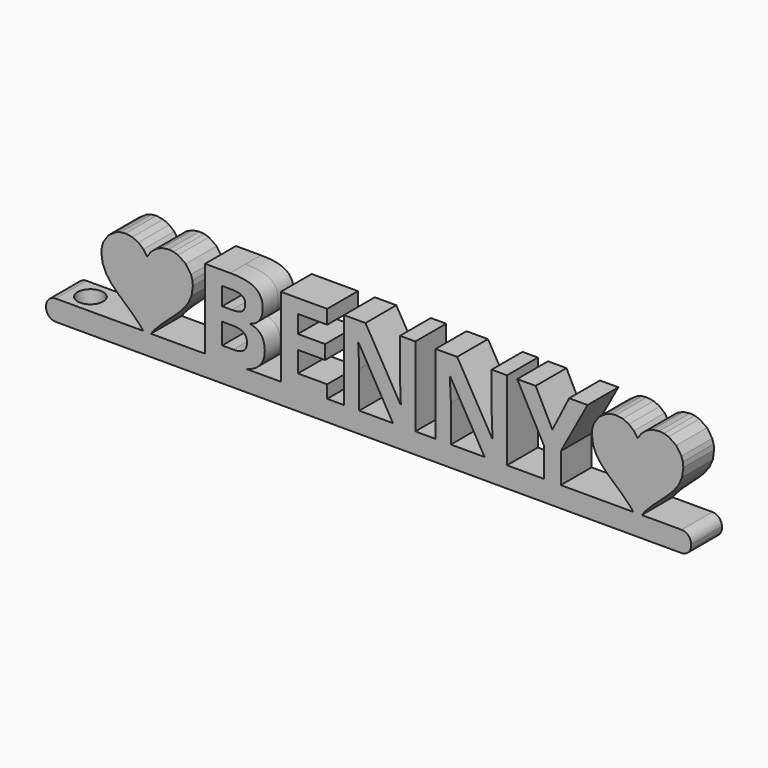
from build123d import *

# Parameters (mm, degrees)
F0_TEXT_SIZE = 17.5671771164
F1_DEPTH     = 3
F2_W         = 93
F2_H         = 6
F3_DEPTH     = 0.2
F4_DEPTH     = 3
F5_W         = 6
F5_H         = 3.2
F6_DEPTH     = 7.5
F7_R         = 1.5
F8_R         = 2
F9_DEPTH     = 4
F10_R        = 1.5


# Not quite as in the source:
# - Text() gives the source's letters only with a copy of the font that has no kerning and outlines rounded to 1/6400 em; it was checked with that copy


with BuildPart() as f1:
    # F0 (on Front) → F1 (new body, symmetric)
    with BuildSketch(Plane.XZ):
        Polygon((61.1623563837, 12.4433699982), (60.1013363837, 12.5970599982), (59.3427263837, 12.5204799982), (58.6359263837, 12.3008699982), (57.4385863837, 11.4933499982), (56.6309663837, 10.2961199982), (56.4113163837, 9.5893599982), (56.3347263837, 8.8307599982), (56.5232463837, 7.3860999982), (57.0439863837, 6.1597099982), (57.8297363837, 5.0814099982), (58.8132663837, 4.0810299982), (61.1101163837, 2.0250499982), (62.2947063837, 0.8247399982), (63.4176963837, -0.5860800018), (63.4619763837, -0.6500000018), (63.5050063837, -0.5851400018), (64.5829163837, 0.8234499982), (65.7462163837, 2.0333299982), (68.0498863837, 4.1212499982), (69.0506763837, 5.1327499982), (69.8556763837, 6.2116199982), (70.3920663837, 7.4226699982), (70.5870463837, 8.8307599982), (70.5104663837, 9.5893599982), (70.2908563837, 10.2961199982), (69.4833363837, 11.4933499982), (68.2861063837, 12.3008699982), (67.5793363837, 12.5204799982), (66.8207463837, 12.5970599982), (65.7597263837, 12.4433699982), (64.8186563837, 12.0123599982), (64.0387063837, 11.3491699982), (63.4610363837, 10.4989199982), (62.8833763837, 11.3491699982), (62.1034263837, 12.0123599982), align=None)
        Polygon((-15.2581707838, 12.5082299799), (-16.3191907838, 12.6619199799), (-17.0778007838, 12.5853399799), (-17.7846007838, 12.3657299799), (-18.9819407838, 11.5582099799), (-19.7895607838, 10.3609799799), (-20.0092107838, 9.6542199799), (-20.0858007838, 8.8956199799), (-19.8972807838, 7.4509599799), (-19.3765407838, 6.2245699799), (-18.5907907838, 5.1462699799), (-17.6072607838, 4.1458899799), (-15.3104107838, 2.0899099799), (-14.1258207838, 0.8895999799), (-13.0028307838, -0.5212200201), (-12.9585507838, -0.5851400201), (-12.9155207838, -0.5202800201), (-11.8376107838, 0.8883099799), (-10.6743107838, 2.0981899799), (-8.3706407838, 4.1861099799), (-7.3698507838, 5.1976099799), (-6.5648507838, 6.2764799799), (-6.0284607838, 7.4875299799), (-5.8334807838, 8.8956199799), (-5.9100607838, 9.6542199799), (-6.1296707838, 10.3609799799), (-6.9371907838, 11.5582099799), (-8.1344207838, 12.3657299799), (-8.8411907838, 12.5853399799), (-9.5997807838, 12.6619199799), (-10.6608007838, 12.5082299799), (-11.6018707838, 12.0772199799), (-12.3818207838, 11.4140299799), (-12.9594907838, 10.5637799799), (-13.5371507838, 11.4140299799), (-14.3171007838, 12.0772199799), align=None)
        with Locations((-5.5058364634, 0)):
            Text('BENNY', F0_TEXT_SIZE, font='Open Sans', font_style=FontStyle.BOLD, text_align=(TextAlign.LEFT, TextAlign.BOTTOM))
    extrude(amount=F1_DEPTH, both=True)



with BuildPart() as f3:
    # F2 (on Top) → F3 (new body)
    with BuildSketch(Plane.XY):
        with Locations((25.3, 0)):
            Rectangle(F2_W, F2_H)
    extrude(amount=F3_DEPTH)


with BuildPart() as f4:
    # F4 (new): a face of the model
    f4_faces = [f3.part.faces().sort_by_distance(p)[0] for p in [
        (25.3, 0, 0),
    ]]
    extrude(f4_faces, amount=F4_DEPTH)


with BuildPart() as f1_1:
    add(f1.part)

    add(f3.part)  # F6 merges F3

    add(f4.part)  # F6 merges F4
    # F5 (on face) → F6 (join)
    with BuildSketch(Plane(origin=(-21.2, 0, 0), x_dir=(0, -1, 0), z_dir=(-1, 0, 0))):
        with Locations((0, -1.4)):
            Rectangle(F5_W, F5_H)
    extrude(amount=F6_DEPTH)

    # F7
    f7_edges = [f1_1.edges().sort_by_distance(p)[0] for p in [
        (-28.7, 0, -3),
        (-28.7, 0, 0.2),
        (71.8, 0, -3),
    ]]
    fillet(f7_edges, radius=F7_R)

    # F8 (on face) → F9 (cut)
    with BuildSketch(Plane.XY.offset(0.2)):
        with Locations((-24.2, 0)):
            Circle(F8_R)
    extrude(amount=-F9_DEPTH, mode=Mode.SUBTRACT)

    # F10
    f10_edges = [f1_1.edges().sort_by_distance(p)[0] for p in [
        (71.8, 0, 0.2),
    ]]
    fillet(f10_edges, radius=F10_R)


solid = f1_1.part
